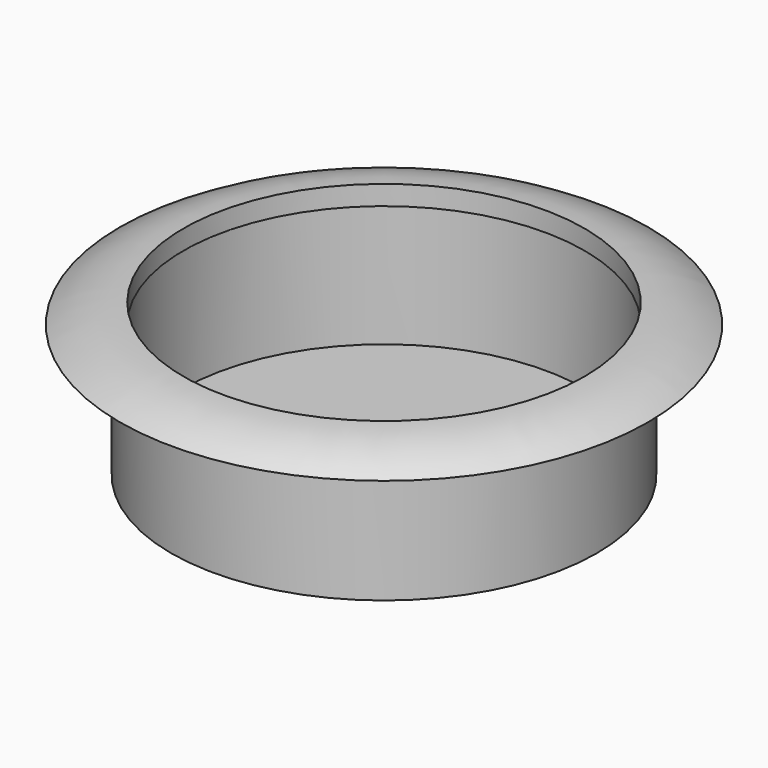
from build123d import *

# Parameters (mm, degrees)
F0_R     = 43.5
F0_R_2   = 41.25
F1_DEPTH = 29
F2_DEPTH = 2
F3_R     = 54
F4_DEPTH = 2
F5_R     = 41
F6_DEPTH = 29.001


# Not quite as in the source:
# - a fillet or chamfer that OpenCascade refuses, or shapes differently, is made with other operations: its cross-section is extruded or revolved along the edge and cut away or added


with BuildPart() as f1:
    # F0 (on Top) → F1 (new body)
    with BuildSketch(Plane.XY):
        Circle(F0_R)
        Circle(F0_R_2, mode=Mode.SUBTRACT)
    extrude(amount=F1_DEPTH)

    # F0 (on Top) → F2 (join)
    with BuildSketch(Plane.XY):
        Circle(F0_R_2)
    extrude(amount=F2_DEPTH)


with BuildPart() as f4:
    # F3 (on face) → F4 (new body, symmetric)
    with BuildSketch(Plane.XY.offset(29)):
        Circle(F3_R)
    extrude(amount=F4_DEPTH, both=True)

    # F5 (on face) → F6 (cut, through all)
    with BuildSketch(Plane.XY.offset(2)):
        Circle(F5_R)
    extrude(amount=F6_DEPTH, mode=Mode.SUBTRACT)

    # F7: fillet of radius 23 on 1 edges, made by hand

    # F7_s1 → F7_t2 (revolve, cut)
    with BuildSketch(Plane.XZ):
        with BuildLine():
            ThreePointArc((54, 27), (47.8208485863, 29.9772609758), (41.0385186032, 31))
            Line((41.0385186032, 31), (41.0385186032, 31.46))
            Line((41.0385186032, 31.46), (54, 31.46))
            Line((54, 31.46), (54.46, 31))
            ThreePointArc((54.46, 31), (54.46, 29), (54.2592296279, 27.38))
            Line((54.2592296279, 27.38), (54, 27))
        make_face()
    revolve(axis=Axis((0, 0, 31), (0, 0, 1)), mode=Mode.SUBTRACT)


solid = Compound([f1.part, f4.part])
